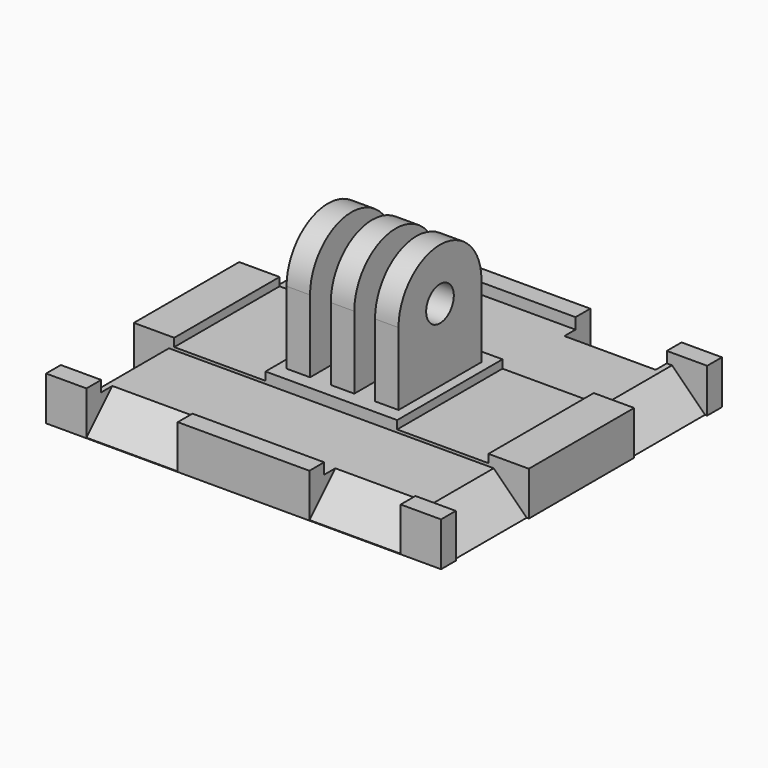
from build123d import *

# Parameters (mm, degrees)
F0_W        = 57.15
F0_H        = 50.8
F1_DEPTH    = 6.35
F2_W        = 13.208
F2_H        = 1.190625
F3_DEPTH    = 50.801
F4_SIZE     = 5.08
F5_W        = 3.4
F5_H        = 15
F6_DEPTH    = 18
F7_W        = 13.208
F7_H        = 1.5875
F8_DEPTH    = 57.151
F9_T1_DEPTH = 13.208
F9_T3_DEPTH = 13.208
F11_D       = 5
F12_DEPTH   = 36.676


# Not quite as in the source:
# - a fillet or chamfer that OpenCascade refuses, or shapes differently, is made with other operations: its cross-section is extruded or revolved along the edge and cut away or added


with BuildPart() as f1:
    # F0 (on Top) → F1 (new body)
    with BuildSketch(Plane.XY):
        Rectangle(F0_W, F0_H)
    extrude(amount=F1_DEPTH)

    # F2 (on face) → F3 (cut, through all)
    with BuildSketch(Plane.XZ.offset(25.4)):
        with Locations((-16.129, 5.7546875)):
            Rectangle(F2_W, F2_H)
        with Locations((16.129, 5.7546875)):
            Rectangle(F2_W, F2_H)
    extrude(amount=-F3_DEPTH, mode=Mode.SUBTRACT)

    # F4
    f4_edges = [f1.edges().sort_by_distance(p)[0] for p in [
        (-16.129, -25.4, 5.159375),
        (16.129, -25.4, 5.159375),
        (-16.129, 25.4, 5.159375),
        (16.129, 25.4, 5.159375),
    ]]
    chamfer(f4_edges, length=F4_SIZE)

    # F5 (on face) → F6 (join)
    with BuildSketch(Plane.XY.offset(6.35)):
        Rectangle(F5_W, F5_H)
        with Locations((6.4, 0)):
            Rectangle(F5_W, F5_H)
        with Locations((-6.4, 0)):
            Rectangle(F5_W, F5_H)
    extrude(amount=F6_DEPTH)

    # F7 (on face) → F8 (cut, through all)
    with BuildSketch(Plane.YZ.offset(28.575)):
        with Locations((-16.129, 5.55625)):
            Rectangle(F7_W, F7_H)
        with Locations((16.129, 5.55625)):
            Rectangle(F7_W, F7_H)
    extrude(amount=-F8_DEPTH, mode=Mode.SUBTRACT)

    # F9: chamfer of 5.08 on 4 edges, made by hand

    # F9_s2 → F9_t1 (cut)
    with BuildSketch(Plane.XZ.offset(-22.733)):
        Polygon((28.575, -0.3175), (23.495, 4.7625), (28.575, 4.7625), align=None)
        Polygon((-28.575, -0.3175), (-23.495, 4.7625), (-28.575, 4.7625), align=None)
    extrude(amount=F9_T1_DEPTH, mode=Mode.SUBTRACT)

    # F9_s4 → F9_t3 (cut)
    with BuildSketch(Plane.XZ.offset(9.525)):
        Polygon((28.575, -0.3175), (23.495, 4.7625), (28.575, 4.7625), align=None)
        Polygon((-28.575, -0.3175), (-23.495, 4.7625), (-28.575, 4.7625), align=None)
    extrude(amount=F9_T3_DEPTH, mode=Mode.SUBTRACT)

    # F11 (through all)
    with Locations(Plane.YZ.offset(8.1)):
        with Locations((0, 16.85)):
            Hole(F11_D / 2)

    # F10 (on face) → F12 (cut, through all)
    with BuildSketch(Plane.YZ.offset(8.1)):
        with BuildLine():
            Line((-7.5, 24.35), (-7.5, 16.85))
            ThreePointArc((-7.5, 16.85), (-5.3033008589, 22.1533008589), (0, 24.35))
            Line((0, 24.35), (-7.5, 24.35))
        make_face()
        with BuildLine():
            Line((7.5, 24.35), (0, 24.35))
            ThreePointArc((0, 24.35), (5.3033008589, 22.1533008589), (7.5, 16.85))
            Line((7.5, 16.85), (7.5, 24.35))
        make_face()
    extrude(amount=-F12_DEPTH, mode=Mode.SUBTRACT)


solid = f1.part
